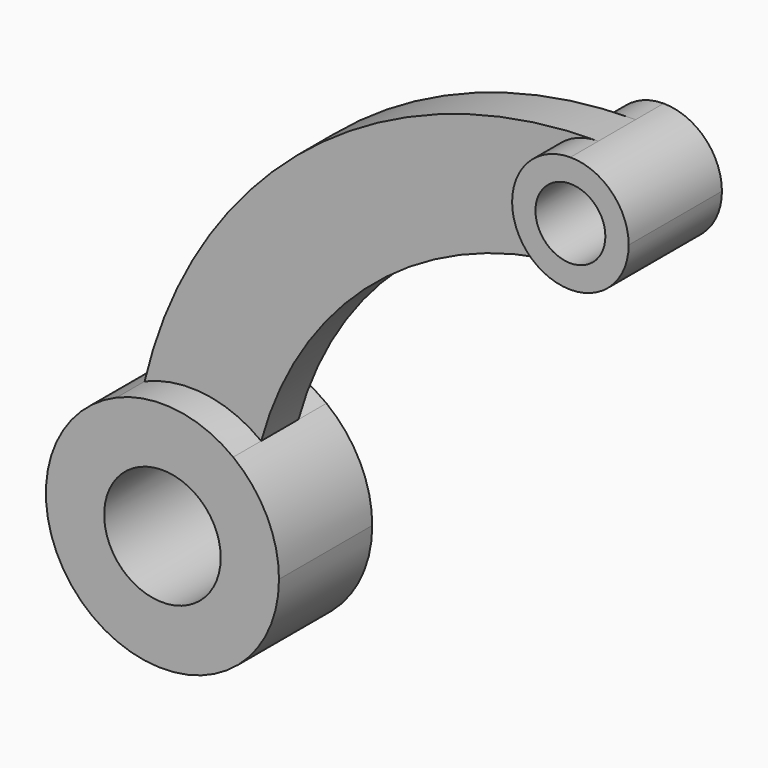
from build123d import *

# Parameters (mm, degrees)
F0_R     = 12.5
F1_DEPTH = 12.5
F0_R_2   = 7.5
F2_DEPTH = 5


with BuildPart() as f1:
    # F0 (on Front) → F1 (new body, symmetric)
    with BuildSketch(Plane.XZ):
        with BuildLine():
            ThreePointArc((-62.5, 0), (-65.089464, 11.080066), (-72.321429, 19.864817))
            ThreePointArc((-72.321429, 19.864817), (-84.398965, 24.806926), (-97.321429, 22.989988))
            ThreePointArc((-97.321429, 22.989988), (-101.274329, -20.863074), (-62.5, 0))
        make_face()
        with Locations((-87.5, 0)):
            Circle(F0_R, mode=Mode.SUBTRACT)
    extrude(amount=F1_DEPTH, both=True)



with BuildPart() as f1b:
    # F0 (on Front) → F1, piece 2 (new body, symmetric)
    with BuildSketch(Plane.XZ):
        with BuildLine():
            ThreePointArc((0, 100), (-12.5, 87.5), (0, 75))
            ThreePointArc((0, 75), (8.838835, 78.661165), (12.5, 87.5))
            ThreePointArc((12.5, 87.5), (8.838835, 96.338835), (0, 100))
        make_face()
        with Locations((0, 87.5)):
            Circle(F0_R_2, mode=Mode.SUBTRACT)
    extrude(amount=F1_DEPTH, both=True)


with BuildPart() as f1_1:
    add(f1.part)

    add(f1b.part)  # F2 merges F1b
    # F0 (on Front) → F2 (join, symmetric)
    with BuildSketch(Plane.XZ):
        with BuildLine():
            ThreePointArc((-72.321429, 19.864817), (-45.470533, 59.6442), (0, 75))
            ThreePointArc((0, 75), (-12.5, 87.5), (0, 100))
            ThreePointArc((0, 100), (-62.052402, 78.418744), (-97.321429, 22.989988))
            ThreePointArc((-97.321429, 22.989988), (-84.398965, 24.806926), (-72.321429, 19.864817))
        make_face()
    extrude(amount=F2_DEPTH, both=True)


solid = f1_1.part
